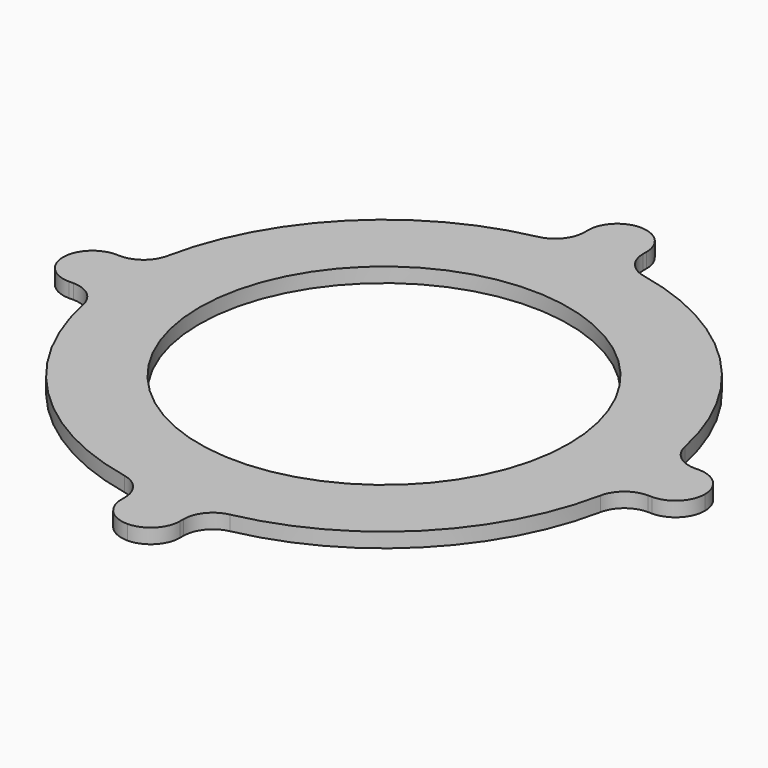
from build123d import *

# Parameters (mm, degrees)
F0_R     = 320.04
F1_DEPTH = 25.4
F2_R     = 50.79999


# Not quite as in the source:
# - a fillet or chamfer is up to 0.001 mm smaller than in the source, because OpenCascade refuses the exact size


with BuildPart() as f1:
    # F0 (on Top) → F1 (new body)
    with BuildSketch(Plane.XY):
        with BuildLine():
            Line((-50.8, 555.969013028), (-50.8, 454.369013028))
            ThreePointArc((-50.8, 454.369013028), (-323.2892203585, 323.2892203585), (-454.369013028, 50.8))
            Line((-454.369013028, 50.8), (-555.969013028, 50.8))
            Line((-555.969013028, 50.8), (-555.969013028, -50.8))
            Line((-555.969013028, -50.8), (-454.369013028, -50.8))
            ThreePointArc((-454.369013028, -50.8), (-323.2892203585, -323.2892203585), (-50.8, -454.369013028))
            Line((-50.8, -454.369013028), (-50.8, -555.969013028))
            Line((-50.8, -555.969013028), (50.8, -555.969013028))
            Line((50.8, -555.969013028), (50.8, -454.369013028))
            ThreePointArc((50.8, -454.369013028), (323.2892203585, -323.2892203585), (454.369013028, -50.8))
            Line((454.369013028, -50.8), (555.969013028, -50.8))
            Line((555.969013028, -50.8), (555.969013028, 50.8))
            Line((555.969013028, 50.8), (454.369013028, 50.8))
            ThreePointArc((454.369013028, 50.8), (323.2892203585, 323.2892203585), (50.8, 454.369013028))
            Line((50.8, 454.369013028), (50.8, 555.969013028))
            Line((50.8, 555.969013028), (-50.8, 555.969013028))
        make_face()
        Circle(F0_R, mode=Mode.SUBTRACT)
    extrude(amount=F1_DEPTH)

    # F2 (radius 50.8 in the source; OpenCascade refuses exactly that, so slightly less here)
    f2_edges = [f1.edges().sort_by_distance(p)[0] for p in [
        (50.8, -555.969013, 12.7),
        (-50.8, -555.969013, 12.7),
        (555.969013, -50.8, 12.7),
        (555.969013, 50.8, 12.7),
        (50.8, 555.969013, 12.7),
        (-50.8, 555.969013, 12.7),
        (-555.969013, 50.8, 12.7),
        (-555.969013, -50.8, 12.7),
        (50.8, -454.369013, 12.7),
        (454.369013, -50.8, 12.7),
        (454.369013, 50.8, 12.7),
        (50.8, 454.369013, 12.7),
        (-50.8, 454.369013, 12.7),
        (-454.369013, 50.8, 12.7),
        (-454.369013, -50.8, 12.7),
        (-50.8, -454.369013, 12.7),
    ]]
    fillet(f2_edges, radius=F2_R)


solid = f1.part
